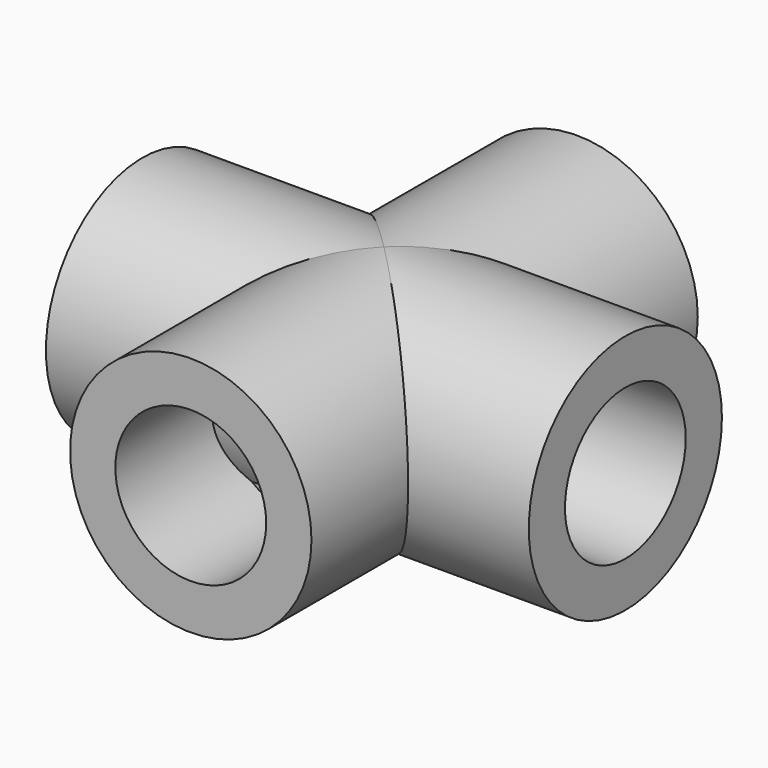
from build123d import *
from build123d import SkipClean  # not in build123d's __all__

# Parameters (mm, degrees)
F0_R     = 31.75
F0_R_2   = 21.59
F1_DEPTH = 44.45
F0_R_3   = 50.8
F2_DEPTH = 101.6
F3_R     = 50.8
F3_R_2   = 31.75
F4_DEPTH = 101.6
F3_R_3   = 21.59
F5_DEPTH = 38.1
F6_DEPTH = 127
F7_DEPTH = 127


with BuildPart() as f1:
    # F0 (on Front) → F1 (new body, symmetric)
    with BuildSketch(Plane.XZ):
        Circle(F0_R)
        Circle(F0_R_2, mode=Mode.SUBTRACT)
    extrude(amount=F1_DEPTH, both=True)

    # F0 (on Front) → F2 (join, symmetric)
    with BuildSketch(Plane.XZ):
        Circle(F0_R_3)
        Circle(F0_R, mode=Mode.SUBTRACT)
    extrude(amount=F2_DEPTH, both=True)



with BuildPart() as f4:
    # F3 (on Right) → F4 (new body, symmetric)
    with BuildSketch(Plane.YZ):
        Circle(F3_R)
        Circle(F3_R_2, mode=Mode.SUBTRACT)
    extrude(amount=F4_DEPTH, both=True)


with BuildPart() as f1_1:
    add(f1.part, clean=False)

    add(f4.part)  # F5 merges F4
    # F3 (on Right) → F5 (join, symmetric)
    with BuildSketch(Plane.YZ):
        Circle(F3_R_2)
        Circle(F3_R_3, mode=Mode.SUBTRACT)
    extrude(amount=F5_DEPTH, both=True)

    # F0 (on Front) → F6 (cut, symmetric)
    with BuildSketch(Plane.XZ):
        Circle(F0_R_2)
    with SkipClean():  # cleaning this boolean's faces spoils the solid; the shape is the same uncleaned
        extrude(amount=F6_DEPTH, both=True, mode=Mode.SUBTRACT)

    # F3 (on Right) → F7 (cut, symmetric)
    with BuildSketch(Plane.YZ):
        Circle(F3_R_3)
    extrude(amount=F7_DEPTH, both=True, mode=Mode.SUBTRACT)


solid = f1_1.part
